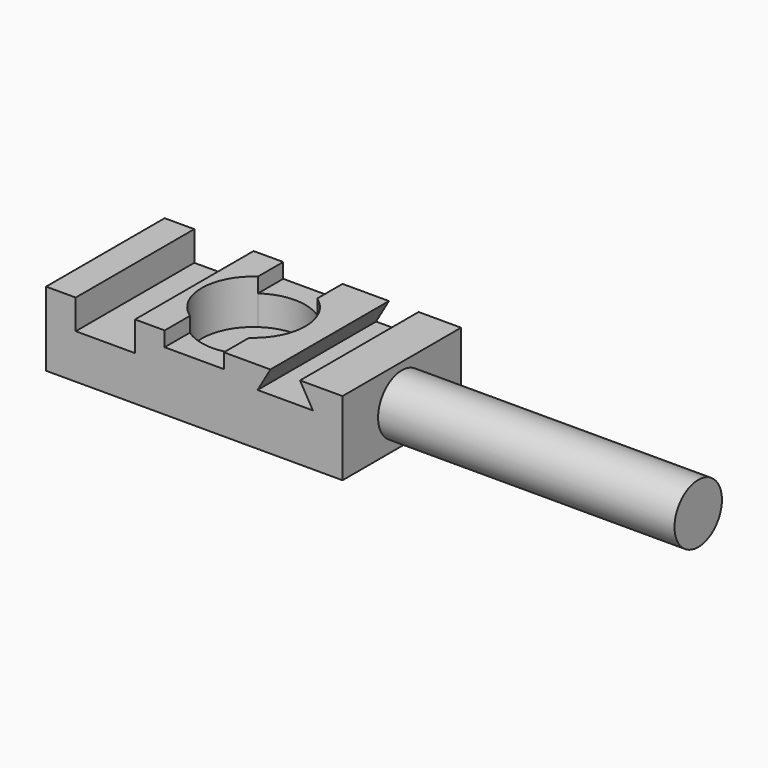
from build123d import *

# Parameters (mm, degrees)
F0_W      = 100
F0_H      = 50
F1_DEPTH  = 25
F2_W      = 20
F2_H      = 50
F3_DEPTH  = 10
F4_DEPTH  = 5
F6_DEPTH  = 50
F7_R      = 10
F8_DEPTH  = 100
F10_DEPTH = 15


# Not quite as in the source:
# - a feature names something its author has since deleted; it is built from what else it names


with BuildPart() as f1:
    # F0 (on Top) → F1 (new body)
    with BuildSketch(Plane.XY):
        Rectangle(F0_W, F0_H)
    extrude(amount=F1_DEPTH)

    # F2 (on face) → F3 (cut)
    with BuildSketch(Plane.XY.offset(25)):
        with Locations((-30, 0)):
            Rectangle(F2_W, F2_H)
    extrude(amount=-F3_DEPTH, mode=Mode.SUBTRACT)

    # F2 (on face) → F4 (cut)
    with BuildSketch(Plane.XY.offset(25)):
        Rectangle(F2_W, F2_H)
    extrude(amount=-F4_DEPTH, mode=Mode.SUBTRACT)

    # F5 (on face) → F6 (cut, through all)
    with BuildSketch(Plane.XZ.offset(25)):
        Polygon((35.6698729811, 25), (25.6698729811, 25), (21.3397459622, 17.5), (40, 17.5), align=None)
    extrude(amount=-F6_DEPTH, mode=Mode.SUBTRACT)

    # F7 (on face) → F8 (join)
    with BuildSketch(Plane.YZ.offset(50)):
        with Locations((0, 12.5)):
            Circle(F7_R)
    extrude(amount=F8_DEPTH)

    # F9 (on face) → F10 (cut)
    with BuildSketch(Plane.XY.offset(25)):
        with BuildLine():
            ThreePointArc((-10, -14.3614066163), (8.100925873, -15.5120920575), (17.5, 0))
            ThreePointArc((17.5, 0), (8.100925873, 15.5120920575), (-10, 14.3614066163))
            Line((-10, 14.3614066163), (-10, -14.3614066163))
        make_face()
        with BuildLine():
            Line((-10, -14.3614066163), (-10, 14.3614066163))
            ThreePointArc((-10, 14.3614066163), (-17.5, 0), (-10, -14.3614066163))
        make_face()
    extrude(amount=-F10_DEPTH, mode=Mode.SUBTRACT)


solid = f1.part
